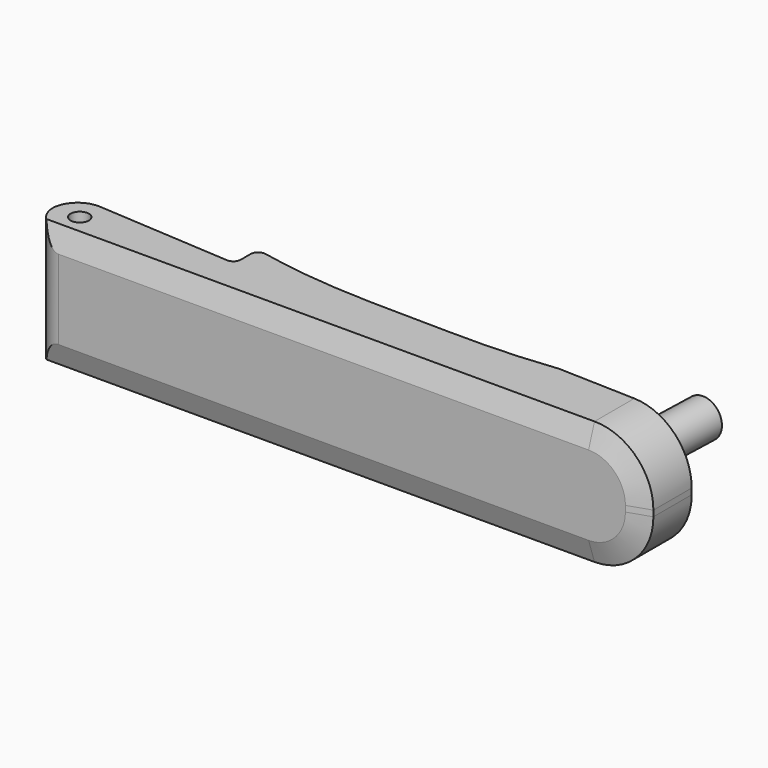
from build123d import *

# Parameters (mm, degrees)
F0_W        = 83.5
F0_H        = 16.8
F1_DEPTH    = 9.5
F2_R        = 1.25
F3_DEPTH    = 25
F4_R        = 2.6
F4_R_2      = 1.05
F5_DEPTH    = 13.6
F6_R        = 1
F7_R        = 8
F8_SIZE2    = 1
F8_SIZE     = 3
F9_T1_DEPTH = 35.4784813046
F9_T3_DEPTH = 40.55


# Not quite as in the source:
# - a fillet or chamfer that OpenCascade refuses, or shapes differently, is made with other operations: its cross-section is extruded or revolved along the edge and cut away or added
# - a feature names something its author has since deleted; it is built from what else it names


with BuildPart() as f1:
    # F0 (on Front) → F1 (new body)
    with BuildSketch(Plane.XZ):
        Rectangle(F0_W, F0_H)
    extrude(amount=F1_DEPTH)

    # F2 (on face) → F3 (cut)
    with BuildSketch(Plane(origin=(0, 0, -8.4), x_dir=(1, 0, 0), z_dir=(0, 0, -1))):
        with Locations((-38.2, 5.95)):
            Circle(F2_R)
        Polygon((-18.75, 0), (-18.75, 4), (-41.75, 2.5), (-41.75, 0), align=None)
        with BuildLine():
            add(Edge.make_bspline(
                [(-18.75, 0), (-9.2352803439, 2.081155549), (4.6071284628, 1.7784279246), (15.029287035, 2.3336862795), (23.25, 1.4)],
                knots=[0, 0, 0, 0, 0.5257635341, 1, 1, 1, 1], degree=3))
            Line((-18.75, 0), (41.75, 0))
            Line((41.75, 0), (41.75, 2))
            Line((41.75, 2), (23.25, 1.4))
        make_face()
    extrude(amount=-F3_DEPTH, mode=Mode.SUBTRACT)

    # F4 (on face) → F5 (join)
    with BuildSketch(Plane(origin=(-0.0209275853, -0.6452672134, 0), x_dir=(-0.9994744832, 0.0324153886, 0), z_dir=(0.0324153886, 0.9994744832, 0))):
        with Locations((-31.7928904511, 0)):
            Circle(F4_R)
        with Locations((-31.7928904511, 0)):
            Circle(F4_R_2, mode=Mode.SUBTRACT)
    extrude(amount=F5_DEPTH)

    # F6
    f6_edges = [f1.edges().sort_by_distance(p)[0] for p in [
        (-18.75, -4, 0),
        (34.353889, -1.760126, 0),
        (-18.75, 0, 0),
    ]]
    fillet(f6_edges, radius=F6_R)

    # F7
    f7_edges = [f1.edges().sort_by_distance(p)[0] for p in [
        (41.75, -5.75, 8.4),
        (41.75, -5.75, -8.4),
    ]]
    fillet(f7_edges, radius=F7_R)

    # F8
    f8_edges = [f1.edges().sort_by_distance(p)[0] for p in [
        (-4, -9.5, 8.4),
    ]]
    f8_side = f1.faces().sort_by_distance((-0.798169, -9.5, 0))[0]
    chamfer(f8_edges, length=F8_SIZE, length2=F8_SIZE2, reference=f8_side)

    # F9: fillet of radius 3.5 on 2 edges, made by hand

    # F9_s2 → F9_t1 (cut)
    with BuildSketch(Plane.XY.offset(-17.7392406523)):
        with BuildLine():
            ThreePointArc((-41.75, -6.2356962609), (-40.6429877316, -3.6815604548), (-38.0222230193, -2.74311589))
            Line((-38.0222230193, -2.74311589), (-41.75, -2.5))
            Line((-41.75, -2.5), (-41.75, -6.2356962609))
        make_face()
    extrude(amount=F9_T1_DEPTH, mode=Mode.SUBTRACT)

    # F9_s4 → F9_t3 (cut)
    with BuildSketch(Plane.XY.offset(-20.275)):
        with BuildLine():
            ThreePointArc((-41.75, -6), (-40.7248737342, -8.4748737342), (-38.25, -9.5))
            Line((-38.25, -9.5), (-41.75, -9.5))
            Line((-41.75, -9.5), (-41.75, -6))
        make_face()
    extrude(amount=F9_T3_DEPTH, mode=Mode.SUBTRACT)


solid = f1.part
